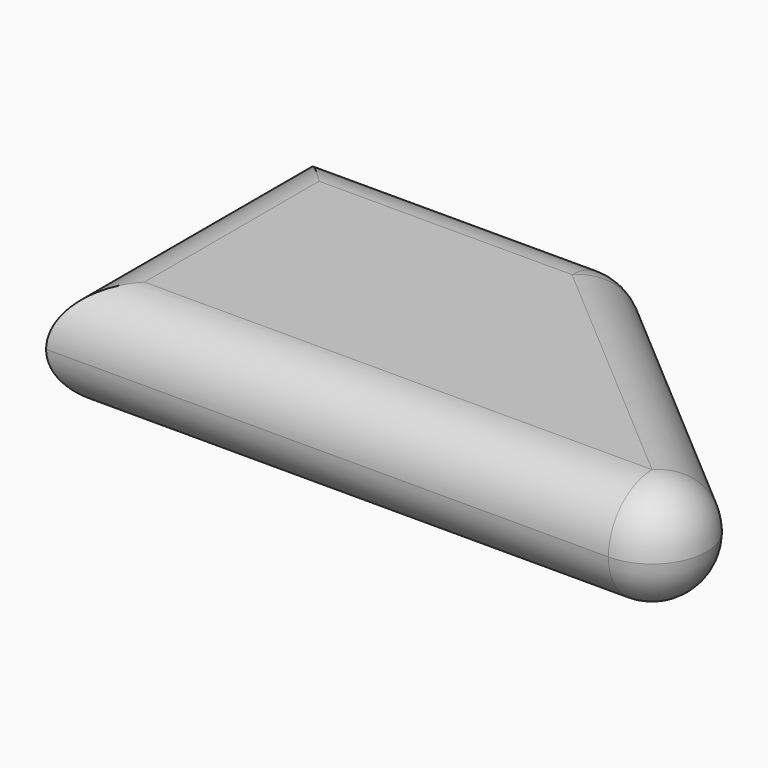
from build123d import *

# Parameters (mm, degrees)
F0_W     = 30
F0_H     = 30
F1_DEPTH = 10
F2_R     = 4.99999


# Not quite as in the source:
# - a fillet or chamfer is up to 0.001 mm smaller than in the source, because OpenCascade refuses the exact size


with BuildPart() as f1:
    # F0 (on Top) → F1 (new body)
    with BuildSketch(Plane.XY):
        Polygon((0, 28.652399919), (-35, 58.652399919), (-35, 28.652399919), align=None)
        with Locations((-50, 43.652399919)):
            Rectangle(F0_W, F0_H)
    extrude(amount=F1_DEPTH)

    # F2 (radius 5 in the source; OpenCascade refuses exactly that, so slightly less here)
    f2_edges = [f1.edges().sort_by_distance(p)[0] for p in [
        (-17.5, 43.6524, 10),
        (-50, 58.6524, 10),
        (-65, 43.6524, 10),
        (-32.5, 28.6524, 10),
        (-32.5, 28.6524, 0),
        (-65, 43.6524, 0),
        (-50, 58.6524, 0),
        (-17.5, 43.6524, 0),
        (-35, 58.6524, 5),
        (0, 28.6524, 5),
    ]]
    fillet(f2_edges, radius=F2_R)


solid = f1.part
